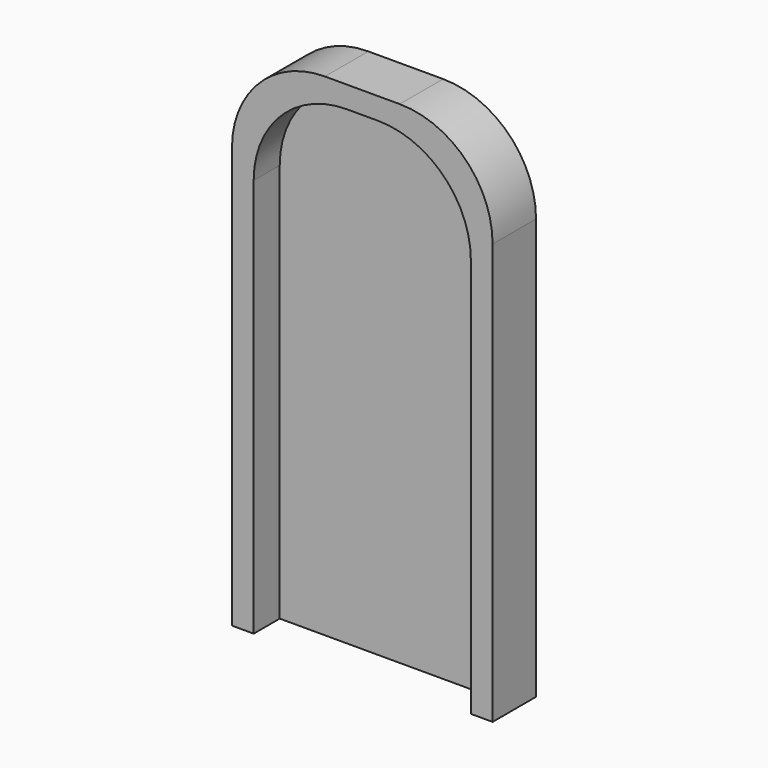
from build123d import *

# Parameters (mm, degrees)
F0_W     = 2.54
F0_H     = 2.54
F1_DEPTH = 6.35
F3_DEPTH = 2.54


# Not quite as in the source:
# - a feature names something its author has since deleted; it is built from what else it names


with BuildPart() as f1:
    # F0 (on Front) → F1 (new body)
    with BuildSketch(Plane.XZ):
        with BuildLine():
            Line((-10.8688886, 57.531), (-10.8688886, 54.991))
            ThreePointArc((-10.8688886, 54.991), (-3.183423767, 51.807576233), (0, 44.1221114))
            Line((0, 44.1221114), (0, 0))
            Line((0, 0), (2.54, 0))
            Line((2.54, 0), (2.54, 46.6621114))
            ThreePointArc((2.54, 46.6621114), (-0.643423767, 54.347576233), (-8.3288886, 57.531))
            Line((-8.3288886, 57.531), (-10.8688886, 57.531))
        make_face()
        with BuildLine():
            Line((-14.5311114, 54.991), (-10.8688886, 54.991))
            Line((-10.8688886, 54.991), (-10.8688886, 57.531))
            Line((-10.8688886, 57.531), (-17.0711114, 57.531))
            ThreePointArc((-17.0711114, 57.531), (-24.756576233, 54.347576233), (-27.94, 46.6621114))
            Line((-27.94, 46.6621114), (-27.94, 0))
            Line((-27.94, 0), (-25.4, 0))
            Line((-25.4, 0), (-25.4, 44.1221114))
            ThreePointArc((-25.4, 44.1221114), (-22.216576233, 51.807576233), (-14.5311114, 54.991))
        make_face()
        with Locations((1.27, -1.27)):
            Rectangle(F0_W, F0_H)
        with Locations((-26.67, -1.27)):
            Rectangle(F0_W, F0_H)
    extrude(amount=F1_DEPTH)

    # F2 (on Front) → F3 (join)
    with BuildSketch(Plane.XZ):
        with BuildLine():
            Line((-27.94, -2.54), (0, -2.54))
            Line((0, -2.54), (2.54, -2.54))
            Line((2.54, -2.54), (2.54, 46.6621114))
            ThreePointArc((2.54, 46.6621114), (-0.643423767, 54.347576233), (-8.3288886, 57.531))
            Line((-8.3288886, 57.531), (-17.0711114, 57.531))
            ThreePointArc((-17.0711114, 57.531), (-24.756576233, 54.347576233), (-27.94, 46.6621114))
            Line((-27.94, 46.6621114), (-27.94, -2.54))
        make_face()
    extrude(amount=F3_DEPTH)


solid = f1.part
